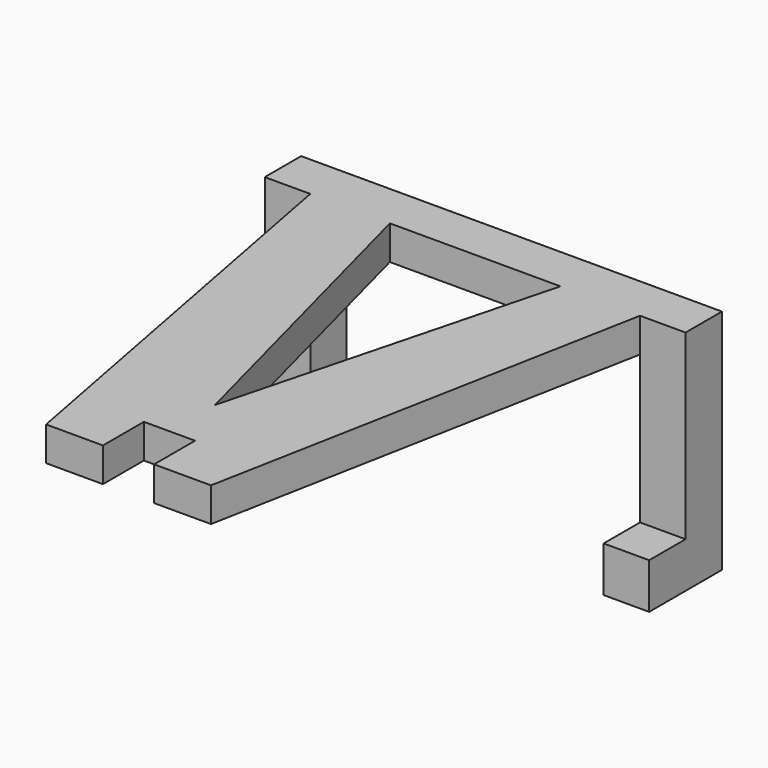
from build123d import *

# Parameters (mm, degrees)
F1_DEPTH = 3
F3_START = 14.5
F2_W     = 4
F2_H     = 13
F3_DEPTH = 4
F6_DEPTH = 25


# Not quite as in the source:
# - a feature names something its author has since deleted; it is built from what else it names


with BuildPart() as f1:
    # F0 (on Top) → F1 (new body)
    with BuildSketch(Plane.XY):
        Polygon((-18.5, 17.05), (-14.5, 17.05), (14.5, 17.05), (18.5, 17.05), (18.5, 21.05), (-18.5, 21.05), align=None)
        Polygon((14.5, 17.05), (-14.5, 17.05), (-7.25, -21.05), (-2.25, -21.05), (-2.25, -16.55), (2.25, -16.55), (2.25, -21.05), (7.25, -21.05), align=None)
    extrude(amount=F1_DEPTH)

    # F2 (on Right) → F3 (join)
    with BuildSketch(Plane.YZ.offset(F3_START)):
        with Locations((19.05, -6.5)):
            Rectangle(F2_W, F2_H)
        Polygon((21.05, -17), (21.05, -13), (17.05, -13), (13.05, -13), (13.05, -17), align=None)
    extrude(amount=F3_DEPTH)

    # F4: F1 across plane


with BuildPart() as f1_1:
    add(f1.part)
    add(f1.part.mirror(Plane.YZ))

    # F5 (on Top) → F6 (cut)
    with BuildSketch(Plane.XY):
        Polygon((7.5, 17.05), (-7.5, 17.05), (0, -11.55), align=None)
    extrude(amount=F6_DEPTH, mode=Mode.SUBTRACT)


solid = f1_1.part
